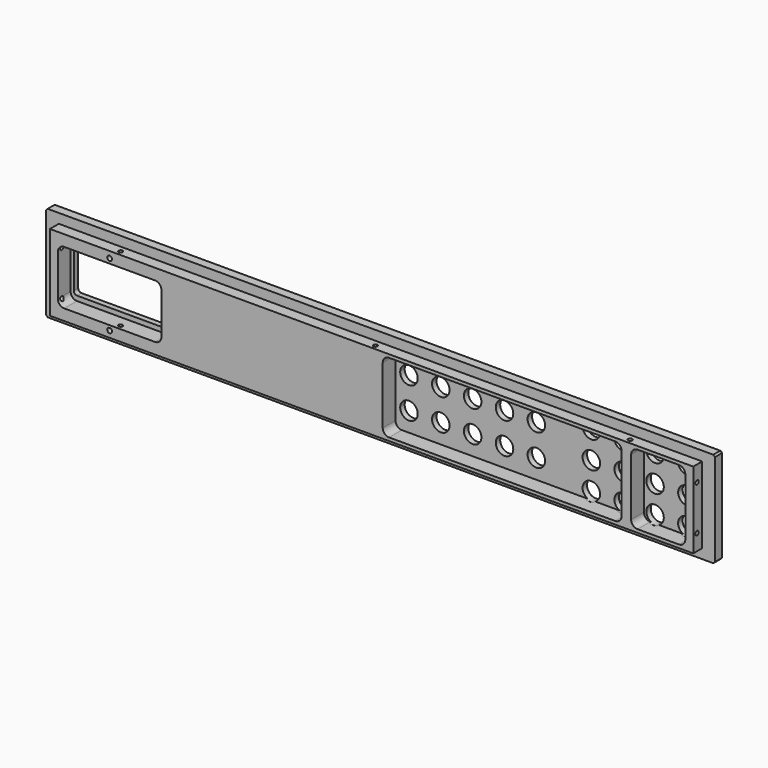
from build123d import *

# Parameters (mm, degrees)
F1_DEPTH      = 210
F0_W          = 7
F0_H          = 48
F2_DEPTH      = 202
F5_D          = 2.6
F5_DEPTH      = 8
F5_TIP        = 0.7811188047
F6_D          = 2.6
F6_DEPTH      = 8
F6_TIP        = 0.7811188047
F9_D          = 2.6
F9_DEPTH      = 6
F9_TIP        = 0.7811188047
F10_D         = 2.6
F10_DEPTH     = 15
F10_TIP       = 0.7811188047
F11_W         = 61
F11_H         = 28
F12_DEPTH     = 12.5
F15_D         = 3
F17_D         = 11
F17_DEPTH     = 5
F17_TIP       = 3.3047334047
F18_D         = 11
F18_DEPTH     = 5
F18_TIP       = 3.3047334047
F19_SIZE      = 1
F20_W         = 65
F20_H         = 34
F20_W_2       = 61
F20_H_2       = 28
F21_DEPTH     = 10
F22_R         = 2
F23_T1_DEPTH  = 10
F23_T6_DEPTH  = 10
F23_S7_R      = 1.3
F23_T8_DEPTH  = 7
F23_T12_DEPTH = 10
F23_S13_R     = 1.3
F23_T14_DEPTH = 7
F20_W_3       = 150
F20_H_3       = 44
F24_DEPTH     = 10
F25_R         = 4
F20_W_4       = 34
F20_H_4       = 43.9752993435
F26_DEPTH     = 10
F27_R         = 4


# Not quite as in the source:
# - a fillet or chamfer that OpenCascade refuses, or shapes differently, is made with other operations: its cross-section is extruded or revolved along the edge and cut away or added
# - a feature names something its author has since deleted; it is built from what else it names


with BuildPart() as f1:
    # F0 (on Right) → F1 (new body, symmetric)
    with BuildSketch(Plane.YZ):
        Polygon((3.25, 30), (-3.25, 30), (-3.25, 24), (-3.25, -24), (-3.25, -30), (3.25, -30), align=None)
    extrude(amount=F1_DEPTH, both=True)

    # F0 (on Right) → F2 (join, symmetric)
    with BuildSketch(Plane.YZ):
        Polygon((3.25, 30), (-3.25, 30), (-3.25, 24), (-3.25, -24), (-3.25, -30), (3.25, -30), align=None)
        with Locations((-6.75, 0)):
            Rectangle(F0_W, F0_H)
    extrude(amount=F2_DEPTH, both=True)

    # F5
    with Locations(Plane.XY.offset(24)):
        with Locations((0, -7.25), (-160, -7.25), (160, -7.25)):
            Hole(F5_D / 2, depth=F5_DEPTH)
            with Locations((0, 0, -(F5_DEPTH + F5_TIP / 2))):  # 118° drill point
                Cone(0, F5_D / 2, F5_TIP, mode=Mode.SUBTRACT)

    # F6
    with Locations(Plane(origin=(0, 0, -24), x_dir=(1, 0, 0), z_dir=(0, 0, -1))):
        with Locations((-160, 7.25), (0, 7.25), (160, 7.25)):
            Hole(F6_D / 2, depth=F6_DEPTH)
            with Locations((0, 0, -(F6_DEPTH + F6_TIP / 2))):  # 118° drill point
                Cone(0, F6_D / 2, F6_TIP, mode=Mode.SUBTRACT)

    # F9
    with Locations(Plane(origin=(-202, 0, 0), x_dir=(0, -1, 0), z_dir=(-1, 0, 0))):
        with Locations((7.25, -14), (7.25, 14)):
            Hole(F9_D / 2, depth=F9_DEPTH)
            with Locations((0, 0, -(F9_DEPTH + F9_TIP / 2))):  # 118° drill point
                Cone(0, F9_D / 2, F9_TIP, mode=Mode.SUBTRACT)

    # F10
    with Locations(Plane.YZ.offset(202)):
        with Locations((-7.25, -14), (-7.25, 14)):
            Hole(F10_D / 2, depth=F10_DEPTH)
            with Locations((0, 0, -(F10_DEPTH + F10_TIP / 2))):  # 118° drill point
                Cone(0, F10_D / 2, F10_TIP, mode=Mode.SUBTRACT)


with BuildPart() as f12:
    # F11 (on Front) → F12 (new body, symmetric)
    with BuildSketch(Plane.XZ):
        with Locations((-164.5, 0)):
            Rectangle(F11_W, F11_H)
    extrude(amount=F12_DEPTH, both=True)


with BuildPart() as f1_1:
    add(f1.part)

    # F13: cut F12
    add(f12.part, mode=Mode.SUBTRACT)

    # F15 (through all)
    with Locations(Plane(origin=(0, 3.25, 0), x_dir=(-1, 0, 0), z_dir=(0, 1, 0))):
        with Locations((164.5, 20), (164.5, -20)):
            Hole(F15_D / 2)

    # F17
    with Locations(Plane(origin=(0, 3.25, 0), x_dir=(-1, 0, 0), z_dir=(0, 1, 0))):
        with Locations((-190, 17), (-170, 17), (-170, 0), (-190, 0), (-75.4730241728, 9.8040188106), (-55.4730241728, 9.8040188106), (-75.4730241728, -9.8040188106), (-55.4730241728, -9.8040188106), (-170, -17), (-190, -17), (-35.4730241728, 9.8040188106), (-15.4730241728, 9.8040188106), (-15.4730241728, -9.8040188106), (-35.4730241728, -9.8040188106), (-150, 17), (-130, 17), (-130, 0), (-150, 0), (-150, -17), (-130, -17)):
            Hole(F17_D / 2, depth=F17_DEPTH)
            with Locations((0, 0, -(F17_DEPTH + F17_TIP / 2))):  # 118° drill point
                Cone(0, F17_D / 2, F17_TIP, mode=Mode.SUBTRACT)

    # F18
    with Locations(Plane(origin=(0, 3.25, 0), x_dir=(-1, 0, 0), z_dir=(0, 1, 0))):
        with Locations((-95.4730241728, -9.8040188106), (-95.4730241728, 9.8040188106)):
            Hole(F18_D / 2, depth=F18_DEPTH)
            with Locations((0, 0, -(F18_DEPTH + F18_TIP / 2))):  # 118° drill point
                Cone(0, F18_D / 2, F18_TIP, mode=Mode.SUBTRACT)

    # F19
    f19_edges = [f1_1.edges().sort_by_distance(p)[0] for p in [
        (210, 0, 30),
        (0, 3.25, 30),
        (210, 3.25, 0),
        (0, 3.25, -30),
        (-210, 3.25, 0),
        (-210, 0, 30),
        (-210, 0, -30),
        (210, 0, -30),
    ]]
    chamfer(f19_edges, length=F19_SIZE)

    # F20 (on face) → F21 (cut, symmetric)
    with BuildSketch(Plane.XZ.offset(10.25)):
        with Locations((-164.5, 0)):
            Rectangle(F20_W, F20_H)
        with Locations((-164.5, 0)):
            Rectangle(F20_W_2, F20_H_2, mode=Mode.SUBTRACT)
    extrude(amount=F21_DEPTH, both=True, mode=Mode.SUBTRACT)

    # F22
    f22_edges = [f1_1.edges().sort_by_distance(p)[0] for p in [
        (-195, 1.5, 14),
        (-134, 1.5, 14),
        (-195, 1.5, -14),
        (-134, 1.5, -14),
    ]]
    fillet(f22_edges, radius=F22_R)

    # F23: fillet of radius 4 on 4 edges, made by hand

    # F23_s2 → F23_t1 (join)
    with BuildSketch(Plane.XZ.offset(0.25)):
        with BuildLine():
            ThreePointArc((-136, 17), (-133.1715728753, 15.8284271247), (-132, 13))
            Line((-132, 13), (-132, 17))
            Line((-132, 17), (-136, 17))
        make_face()
        with BuildLine():
            ThreePointArc((-136, -17), (-133.1715728753, -15.8284271247), (-132, -13))
            Line((-132, -13), (-132, -17))
            Line((-132, -17), (-136, -17))
        make_face()
    extrude(amount=F23_T1_DEPTH)


with BuildPart() as f23_tool4:
    # F23_s5 → F23_t6 (new body)
    with BuildSketch(Plane.XZ.offset(0.25)):
        with BuildLine():
            ThreePointArc((-193, 17), (-195.8284271247, 15.8284271247), (-197, 13))
            Line((-197, 13), (-197, 17))
            Line((-197, 17), (-193, 17))
        make_face()
    extrude(amount=F23_T6_DEPTH)

    # F23_s7 → F23_t8 (cut, symmetric)
    with BuildSketch(Plane.YZ.offset(-195)):
        with Locations((-7.25, 14)):
            Circle(F23_S7_R)
    extrude(amount=F23_T8_DEPTH, both=True, mode=Mode.SUBTRACT)


with BuildPart() as f1_2:
    add(f1_1.part)

    # F23_t3: union F23_tool4
    add(f23_tool4.part)


with BuildPart() as f23_tool10:
    # F23_s11 → F23_t12 (new body)
    with BuildSketch(Plane.XZ.offset(0.25)):
        with BuildLine():
            ThreePointArc((-197, -13), (-195.8284271247, -15.8284271247), (-193, -17))
            Line((-193, -17), (-197, -17))
            Line((-197, -17), (-197, -13))
        make_face()
    extrude(amount=F23_T12_DEPTH)

    # F23_s13 → F23_t14 (cut, symmetric)
    with BuildSketch(Plane.YZ.offset(-195)):
        with Locations((-7.25, -14)):
            Circle(F23_S13_R)
    extrude(amount=F23_T14_DEPTH, both=True, mode=Mode.SUBTRACT)


with BuildPart() as f1_3:
    add(f1_2.part)

    # F23_t9: union F23_tool10
    add(f23_tool10.part)

    # F20 (on face) → F24 (cut, symmetric)
    with BuildSketch(Plane.XZ.offset(10.25)):
        with Locations((82, 0)):
            Rectangle(F20_W_3, F20_H_3)
    extrude(amount=F24_DEPTH, both=True, mode=Mode.SUBTRACT)

    # F25
    f25_edges = [f1_3.edges().sort_by_distance(p)[0] for p in [
        (157, -5.25, 22),
        (157, -5.25, -22),
        (7, -5.25, -22),
        (7, -5.25, 22),
    ]]
    fillet(f25_edges, radius=F25_R)

    # F20 (on face) → F26 (cut, symmetric)
    with BuildSketch(Plane.XZ.offset(10.25)):
        with Locations((180, 0.0123503283)):
            Rectangle(F20_W_4, F20_H_4)
    extrude(amount=F26_DEPTH, both=True, mode=Mode.SUBTRACT)

    # F27
    f27_edges = [f1_3.edges().sort_by_distance(p)[0] for p in [
        (163, -5.25, -21.975299),
        (163, -5.25, 22),
        (197, -5.25, 22),
        (197, -5.25, -21.975299),
    ]]
    fillet(f27_edges, radius=F27_R)


solid = f1_3.part
